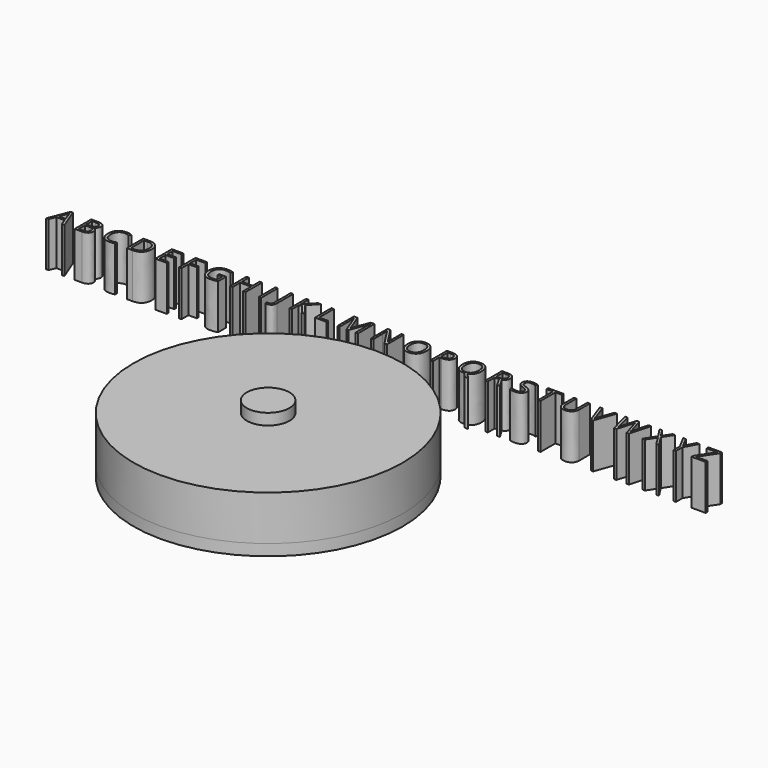
from build123d import *

# Parameters (mm, degrees)
F0_R           = 12.065
F1_DEPTH       = 31.75
F1_DEPTH_BACK  = 6.35
F2_R           = 76.2
F3_DEPTH       = 6.35
F4_D           = 12.7
F4_CSINK_D     = 25.4
F4_CSINK_ANGLE = 90
F5_SIZE2       = 6.34999
F5_SIZE        = 6.34999
F6_R           = 76.2
F6_TEXT_SIZE   = 16.36334281
F7_DEPTH       = 25.4


# Not quite as in the source:
# - a fillet or chamfer is up to 0.001 mm smaller than in the source, because OpenCascade refuses the exact size
# - Text() gives the source's letters only with a copy of the font that has no kerning and outlines rounded to 1/6400 em; it was checked with that copy


with BuildPart() as f1:
    # F0 (on Top) → F1 (new body, two sides)
    with BuildSketch(Plane.XY) as f1_sk:
        Circle(F0_R)
    extrude(amount=F1_DEPTH)
    extrude(f1_sk.sketch, amount=-F1_DEPTH_BACK)

    # F5 (size 6.35 and 6.35 in the source; OpenCascade refuses exactly that, so slightly less here)
    f5_edges = [f1.edges().sort_by_distance(p)[0] for p in [
        (-12.065, 0, -6.35),
    ]]
    chamfer(f5_edges, length=F5_SIZE, length2=F5_SIZE2)


with BuildPart() as f3:
    # F2 (on face) → F3 (new body)
    with BuildSketch(Plane(origin=(0, 0, -6.35), x_dir=(1, 0, 0), z_dir=(0, 0, -1))):
        Circle(F2_R)
    extrude(amount=-F3_DEPTH)

    # F4 (through all)
    with Locations(Plane.XY):
        with Locations((0, 0)):
            CounterSinkHole(F4_D / 2, F4_CSINK_D / 2, counter_sink_angle=F4_CSINK_ANGLE)


with BuildPart() as f7:
    # F6 (on Top) → F7 (new body)
    with BuildSketch(Plane.XY):
        Circle(F6_R)
        with Locations((-192.9384344257, 84.1233264655)):
            Text('A B C D E F G H I J K L M N O P Q R S T U V W X Y Z', F6_TEXT_SIZE, font='Open Sans', text_align=(TextAlign.LEFT, TextAlign.BOTTOM))
    extrude(amount=F7_DEPTH)


solid = Compound([f1.part, f3.part, f7.part])
